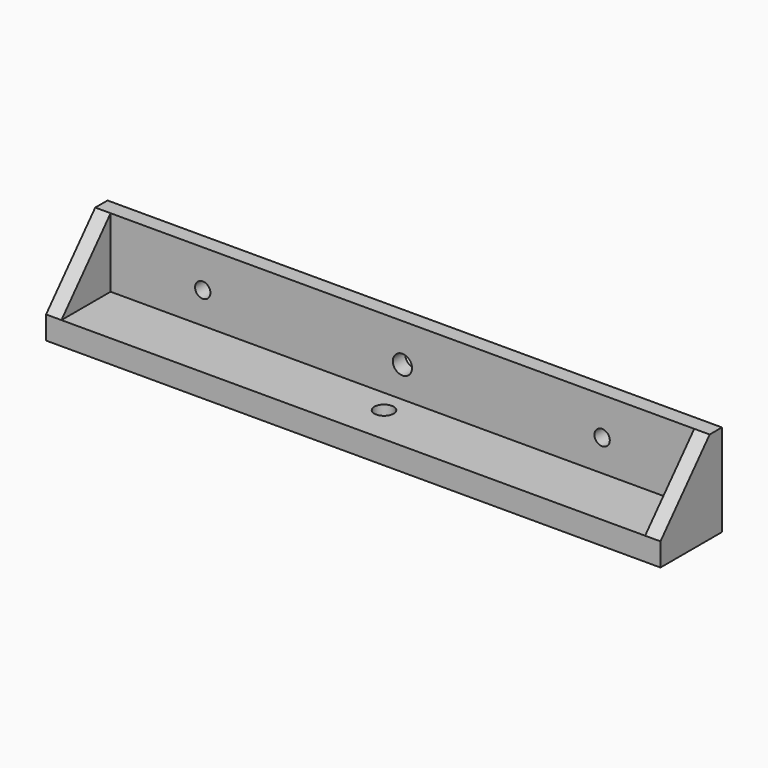
from build123d import *

# Parameters (mm, degrees)
F0_W      = 80
F0_H      = 10
F1_DEPTH  = 3
F2_W      = 80
F2_H      = 2
F3_DEPTH  = 9
F4_R      = 1.25
F5_DEPTH  = 3.001
F6_R      = 1.25
F7_DEPTH  = 2.001
F9_DEPTH  = 2
F10_R     = 1
F11_DEPTH = 2.001


# Not quite as in the source:
# - a pattern or mirror of a feature is missing from the dataset's text; its kind, count and spacing are read off the source's solid


with BuildPart() as f1:
    # F0 (on Top) → F1 (new body)
    with BuildSketch(Plane.XY):
        Rectangle(F0_W, F0_H)
    extrude(amount=F1_DEPTH)

    # F2 (on face) → F3 (join)
    with BuildSketch(Plane.XY.offset(3)):
        with Locations((0, 4)):
            Rectangle(F2_W, F2_H)
    extrude(amount=F3_DEPTH)

    # F4 (on face) → F5 (cut, through all)
    with BuildSketch(Plane.XY.offset(3)):
        Circle(F4_R)
    extrude(amount=-F5_DEPTH, mode=Mode.SUBTRACT)

    # F6 (on face) → F7 (cut, through all)
    with BuildSketch(Plane.XZ.offset(-3)):
        with Locations((0, 7)):
            Circle(F6_R)
    extrude(amount=-F7_DEPTH, mode=Mode.SUBTRACT)

    # F8 (on face) → F9 (join)
    with BuildSketch(Plane(origin=(-40, 0, 0), x_dir=(0, -1, 0), z_dir=(-1, 0, 0))):
        Polygon((5, 3), (-3, 12), (-3, 3), align=None)
    f9 = extrude(amount=-F9_DEPTH)

    # F9_copies: F9 across plane
    add(f9.mirror(Plane(origin=(0, 0, 0), x_dir=(0, 0, 1), z_dir=(1, 0, 0))))

    # F10 (on face) → F11 (cut, through all)
    with BuildSketch(Plane.XZ.offset(-3)):
        with Locations((-26, 7.0934407413)):
            Circle(F10_R)
        with Locations((26, 7.0934407413)):
            Circle(F10_R)
    extrude(amount=-F11_DEPTH, mode=Mode.SUBTRACT)


solid = f1.part
